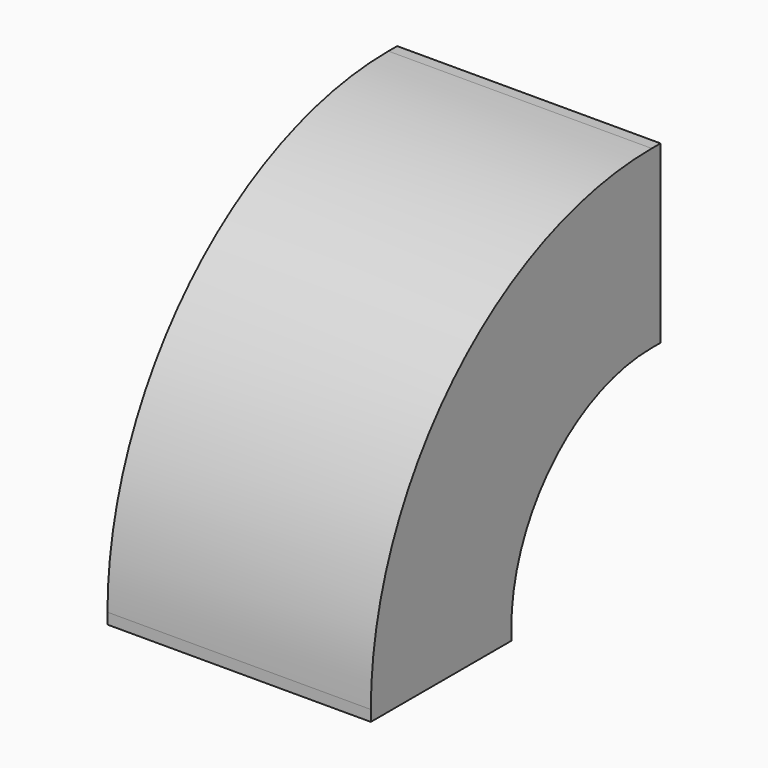
from build123d import *

# Parameters (mm, degrees)
F0_W     = 914.4
F0_H     = 609.6
F1_DEPTH = 38.1
F2_W     = 914.4
F2_H     = 609.6
F3_ANGLE = 90
F4_DEPTH = 38.1


with BuildPart() as f1:
    # F0 (on Top) → F1 (new body)
    with BuildSketch(Plane.XY):
        Rectangle(F0_W, F0_H)
    extrude(amount=F1_DEPTH)

    # F2 (on face) → F3 (revolve)
    with BuildSketch(Plane.XY.offset(38.1)):
        Rectangle(F2_W, F2_H)
    revolve(axis=Axis((-103.2055318356, 914.4, 38.1), (-1, 0, 0)), revolution_arc=F3_ANGLE)

    # F4 (add): a face of the model
    f4_faces = [f1.faces().sort_by_distance(p)[0] for p in [
        (0, 914.4, 952.5),
    ]]
    extrude(f4_faces, amount=F4_DEPTH)


solid = f1.part
